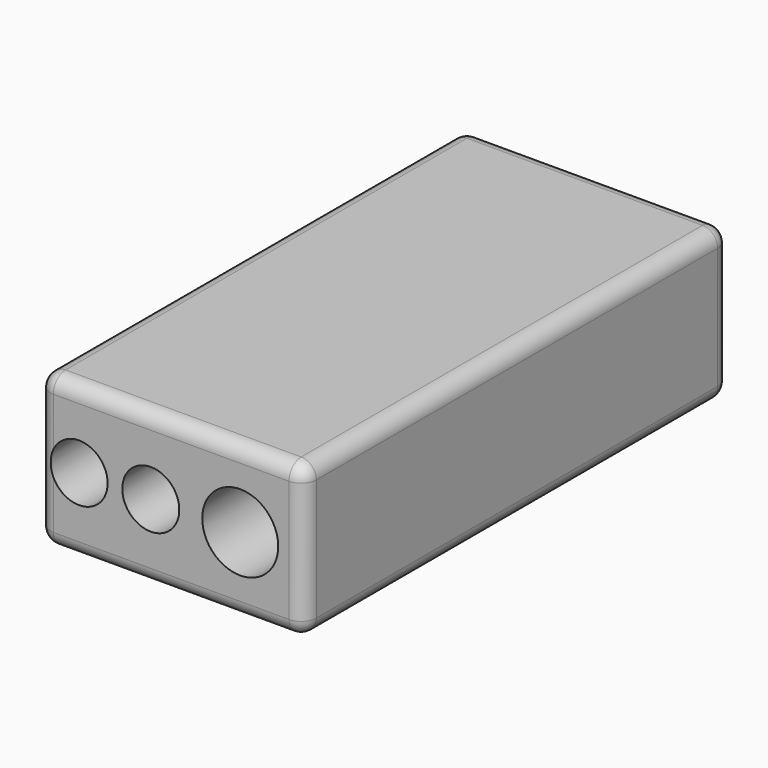
from build123d import *

# Parameters (mm, degrees)
F0_W         = 88.9
F0_H         = 50.8
F1_DEPTH     = 177.8
F3_D         = 19.05
F5_D         = 25.4
F6_T1_DEPTH  = 167.64
F6_T3_DEPTH  = 78.74
F6_T5_DEPTH  = 40.64
F6_S9_W      = 5.08
F6_S9_H      = 5.08
F6_T10_DEPTH = 5.08
F6_S15_W     = 5.08
F6_S15_H     = 5.08
F6_T16_DEPTH = 5.08
F6_S21_W     = 5.08
F6_S21_H     = 5.08
F6_T22_DEPTH = 5.08
F6_S27_W     = 5.08
F6_S27_H     = 5.08
F6_T28_DEPTH = 5.08
F6_S33_W     = 5.08
F6_S33_H     = 5.08
F6_T34_DEPTH = 5.08
F6_S39_W     = 5.08
F6_S39_H     = 5.08
F6_T40_DEPTH = 5.08
F6_S45_W     = 5.08
F6_S45_H     = 5.08
F6_T46_DEPTH = 5.08
F6_S51_W     = 5.08
F6_S51_H     = 5.08
F6_T52_DEPTH = 5.08


# Not quite as in the source:
# - a fillet or chamfer that OpenCascade refuses, or shapes differently, is made with other operations: its cross-section is extruded or revolved along the edge and cut away or added


with BuildPart() as f1:
    # F0 (on Front) → F1 (new body)
    with BuildSketch(Plane.XZ):
        Rectangle(F0_W, F0_H)
    extrude(amount=F1_DEPTH)

    # F3 (through all)
    with Locations(Plane.XZ.offset(177.8)):
        with Locations((-30.7692382485, 0), (-6.8131890148, 0)):
            Hole(F3_D / 2)

    # F5 (through all)
    with Locations(Plane(origin=(0, 0, 0), x_dir=(1, 0, 0), z_dir=(0, 1, 0))):
        with Locations((23.0769272894, 0)):
            Hole(F5_D / 2)

    # F6: fillet of radius 5.08 on 12 edges, made by hand

    # F6_s2 → F6_t1 (cut)
    with BuildSketch(Plane.XZ.offset(5.08)):
        with BuildLine():
            ThreePointArc((44.45, 20.32), (42.9621024484, 23.9121024484), (39.37, 25.4))
            Line((39.37, 25.4), (44.45, 25.4))
            Line((44.45, 25.4), (44.45, 20.32))
        make_face()
        with BuildLine():
            ThreePointArc((-44.45, 20.32), (-42.9621024484, 23.9121024484), (-39.37, 25.4))
            Line((-39.37, 25.4), (-44.45, 25.4))
            Line((-44.45, 25.4), (-44.45, 20.32))
        make_face()
        with BuildLine():
            ThreePointArc((39.37, -25.4), (42.9621024484, -23.9121024484), (44.45, -20.32))
            Line((44.45, -20.32), (44.45, -25.4))
            Line((44.45, -25.4), (39.37, -25.4))
        make_face()
        with BuildLine():
            ThreePointArc((-39.37, -25.4), (-42.9621024484, -23.9121024484), (-44.45, -20.32))
            Line((-44.45, -20.32), (-44.45, -25.4))
            Line((-44.45, -25.4), (-39.37, -25.4))
        make_face()
    extrude(amount=F6_T1_DEPTH, mode=Mode.SUBTRACT)

    # F6_s4 → F6_t3 (cut)
    with BuildSketch(Plane.YZ.offset(-39.37)):
        with BuildLine():
            ThreePointArc((0, 20.32), (-1.4878975516, 23.9121024484), (-5.08, 25.4))
            Line((-5.08, 25.4), (0, 25.4))
            Line((0, 25.4), (0, 20.32))
        make_face()
        with BuildLine():
            ThreePointArc((-177.8, 20.32), (-176.3121024484, 23.9121024484), (-172.72, 25.4))
            Line((-172.72, 25.4), (-177.8, 25.4))
            Line((-177.8, 25.4), (-177.8, 20.32))
        make_face()
        with BuildLine():
            ThreePointArc((-5.08, -25.4), (-1.4878975516, -23.9121024484), (0, -20.32))
            Line((0, -20.32), (0, -25.4))
            Line((0, -25.4), (-5.08, -25.4))
        make_face()
        with BuildLine():
            ThreePointArc((-172.72, -25.4), (-176.3121024484, -23.9121024484), (-177.8, -20.32))
            Line((-177.8, -20.32), (-177.8, -25.4))
            Line((-177.8, -25.4), (-172.72, -25.4))
        make_face()
    extrude(amount=F6_T3_DEPTH, mode=Mode.SUBTRACT)

    # F6_s6 → F6_t5 (cut)
    with BuildSketch(Plane.XY.offset(-20.32)):
        with BuildLine():
            ThreePointArc((44.45, -5.08), (42.9621024484, -1.4878975516), (39.37, 0))
            Line((39.37, 0), (44.45, 0))
            Line((44.45, 0), (44.45, -5.08))
        make_face()
        with BuildLine():
            ThreePointArc((44.45, -172.72), (42.9621024484, -176.3121024484), (39.37, -177.8))
            Line((39.37, -177.8), (44.45, -177.8))
            Line((44.45, -177.8), (44.45, -172.72))
        make_face()
        with BuildLine():
            ThreePointArc((-44.45, -5.08), (-42.9621024484, -1.4878975516), (-39.37, 0))
            Line((-39.37, 0), (-44.45, 0))
            Line((-44.45, 0), (-44.45, -5.08))
        make_face()
        with BuildLine():
            ThreePointArc((-44.45, -172.72), (-42.9621024484, -176.3121024484), (-39.37, -177.8))
            Line((-39.37, -177.8), (-44.45, -177.8))
            Line((-44.45, -177.8), (-44.45, -172.72))
        make_face()
    extrude(amount=F6_T5_DEPTH, mode=Mode.SUBTRACT)


with BuildPart() as f6_tool8:
    # F6_s9 → F6_t10 (new body)
    with BuildSketch(Plane.YZ.offset(39.37)):
        with Locations((-2.54, 22.86)):
            Rectangle(F6_S9_W, F6_S9_H)
    extrude(amount=F6_T10_DEPTH)

    # F6_s11 → F6_t12 (revolve, cut)
    with BuildSketch(Plane(origin=(39.37, -5.08, 20.32), x_dir=(0, -0.7071067812, -0.7071067812), z_dir=(0, -0.7071067812, 0.7071067812))):
        with BuildLine():
            ThreePointArc((0, -5.08), (5.08, 0), (0, 5.08))
            Line((0, 5.08), (0, -5.08))
        make_face()
    revolve(axis=Axis((39.37, -5.08, 20.32), (1, 0, 0)), mode=Mode.SUBTRACT)


with BuildPart() as f1_1:
    add(f1.part)

    # F6_t7: cut F6_tool8
    add(f6_tool8.part, mode=Mode.SUBTRACT)


with BuildPart() as f6_tool14:
    # F6_s15 → F6_t16 (new body)
    with BuildSketch(Plane.YZ.offset(39.37)):
        with Locations((-175.26, 22.86)):
            Rectangle(F6_S15_W, F6_S15_H)
    extrude(amount=F6_T16_DEPTH)

    # F6_s17 → F6_t18 (revolve, cut)
    with BuildSketch(Plane(origin=(39.37, -172.72, 20.32), x_dir=(0, 0.7071067812, -0.7071067812), z_dir=(0, -0.7071067812, -0.7071067812))):
        with BuildLine():
            ThreePointArc((0, -5.08), (5.08, 0), (0, 5.08))
            Line((0, 5.08), (0, -5.08))
        make_face()
    revolve(axis=Axis((39.37, -172.72, 20.32), (1, 0, 0)), mode=Mode.SUBTRACT)


with BuildPart() as f1_2:
    add(f1_1.part)

    # F6_t13: cut F6_tool14
    add(f6_tool14.part, mode=Mode.SUBTRACT)


with BuildPart() as f6_tool20:
    # F6_s21 → F6_t22 (new body)
    with BuildSketch(Plane.YZ.offset(-39.37)):
        with Locations((-2.54, 22.86)):
            Rectangle(F6_S21_W, F6_S21_H)
    extrude(amount=-F6_T22_DEPTH)

    # F6_s23 → F6_t24 (revolve, cut)
    with BuildSketch(Plane(origin=(-39.37, -5.08, 20.32), x_dir=(0, -0.7071067812, -0.7071067812), z_dir=(0, 0.7071067812, -0.7071067812))):
        with BuildLine():
            ThreePointArc((0, -5.08), (5.08, 0), (0, 5.08))
            Line((0, 5.08), (0, -5.08))
        make_face()
    revolve(axis=Axis((-39.37, -5.08, 20.32), (-1, 0, 0)), mode=Mode.SUBTRACT)


with BuildPart() as f1_3:
    add(f1_2.part)

    # F6_t19: cut F6_tool20
    add(f6_tool20.part, mode=Mode.SUBTRACT)


with BuildPart() as f6_tool26:
    # F6_s27 → F6_t28 (new body)
    with BuildSketch(Plane.YZ.offset(-39.37)):
        with Locations((-175.26, 22.86)):
            Rectangle(F6_S27_W, F6_S27_H)
    extrude(amount=-F6_T28_DEPTH)

    # F6_s29 → F6_t30 (revolve, cut)
    with BuildSketch(Plane(origin=(-39.37, -172.72, 20.32), x_dir=(0, 0.7071067812, -0.7071067812), z_dir=(0, 0.7071067812, 0.7071067812))):
        with BuildLine():
            ThreePointArc((0, -5.08), (5.08, 0), (0, 5.08))
            Line((0, 5.08), (0, -5.08))
        make_face()
    revolve(axis=Axis((-39.37, -172.72, 20.32), (-1, 0, 0)), mode=Mode.SUBTRACT)


with BuildPart() as f1_4:
    add(f1_3.part)

    # F6_t25: cut F6_tool26
    add(f6_tool26.part, mode=Mode.SUBTRACT)


with BuildPart() as f6_tool32:
    # F6_s33 → F6_t34 (new body)
    with BuildSketch(Plane.XY.offset(-20.32)):
        with Locations((41.91, -2.54)):
            Rectangle(F6_S33_W, F6_S33_H)
    extrude(amount=-F6_T34_DEPTH)

    # F6_s35 → F6_t36 (revolve, cut)
    with BuildSketch(Plane(origin=(39.37, -5.08, -20.32), x_dir=(-0.7071067812, -0.7071067812, 0), z_dir=(0.7071067812, -0.7071067812, 0))):
        with BuildLine():
            ThreePointArc((0, -5.08), (5.08, 0), (0, 5.08))
            Line((0, 5.08), (0, -5.08))
        make_face()
    revolve(axis=Axis((39.37, -5.08, -20.32), (0, 0, -1)), mode=Mode.SUBTRACT)


with BuildPart() as f1_5:
    add(f1_4.part)

    # F6_t31: cut F6_tool32
    add(f6_tool32.part, mode=Mode.SUBTRACT)


with BuildPart() as f6_tool38:
    # F6_s39 → F6_t40 (new body)
    with BuildSketch(Plane.XY.offset(-20.32)):
        with Locations((41.91, -175.26)):
            Rectangle(F6_S39_W, F6_S39_H)
    extrude(amount=-F6_T40_DEPTH)

    # F6_s41 → F6_t42 (revolve, cut)
    with BuildSketch(Plane(origin=(39.37, -172.72, -20.32), x_dir=(-0.7071067812, 0.7071067812, 0), z_dir=(-0.7071067812, -0.7071067812, 0))):
        with BuildLine():
            ThreePointArc((0, -5.08), (5.08, 0), (0, 5.08))
            Line((0, 5.08), (0, -5.08))
        make_face()
    revolve(axis=Axis((39.37, -172.72, -20.32), (0, 0, -1)), mode=Mode.SUBTRACT)


with BuildPart() as f1_6:
    add(f1_5.part)

    # F6_t37: cut F6_tool38
    add(f6_tool38.part, mode=Mode.SUBTRACT)


with BuildPart() as f6_tool44:
    # F6_s45 → F6_t46 (new body)
    with BuildSketch(Plane.XY.offset(-20.32)):
        with Locations((-41.91, -2.54)):
            Rectangle(F6_S45_W, F6_S45_H)
    extrude(amount=-F6_T46_DEPTH)

    # F6_s47 → F6_t48 (revolve, cut)
    with BuildSketch(Plane(origin=(-39.37, -5.08, -20.32), x_dir=(0.7071067812, -0.7071067812, 0), z_dir=(0.7071067812, 0.7071067812, 0))):
        with BuildLine():
            ThreePointArc((0, -5.08), (5.08, 0), (0, 5.08))
            Line((0, 5.08), (0, -5.08))
        make_face()
    revolve(axis=Axis((-39.37, -5.08, -20.32), (0, 0, -1)), mode=Mode.SUBTRACT)


with BuildPart() as f1_7:
    add(f1_6.part)

    # F6_t43: cut F6_tool44
    add(f6_tool44.part, mode=Mode.SUBTRACT)


with BuildPart() as f6_tool50:
    # F6_s51 → F6_t52 (new body)
    with BuildSketch(Plane.XY.offset(-20.32)):
        with Locations((-41.91, -175.26)):
            Rectangle(F6_S51_W, F6_S51_H)
    extrude(amount=-F6_T52_DEPTH)

    # F6_s53 → F6_t54 (revolve, cut)
    with BuildSketch(Plane(origin=(-39.37, -172.72, -20.32), x_dir=(0.7071067812, 0.7071067812, 0), z_dir=(-0.7071067812, 0.7071067812, 0))):
        with BuildLine():
            ThreePointArc((0, -5.08), (5.08, 0), (0, 5.08))
            Line((0, 5.08), (0, -5.08))
        make_face()
    revolve(axis=Axis((-39.37, -172.72, -20.32), (0, 0, -1)), mode=Mode.SUBTRACT)


with BuildPart() as f1_8:
    add(f1_7.part)

    # F6_t49: cut F6_tool50
    add(f6_tool50.part, mode=Mode.SUBTRACT)


solid = f1_8.part
